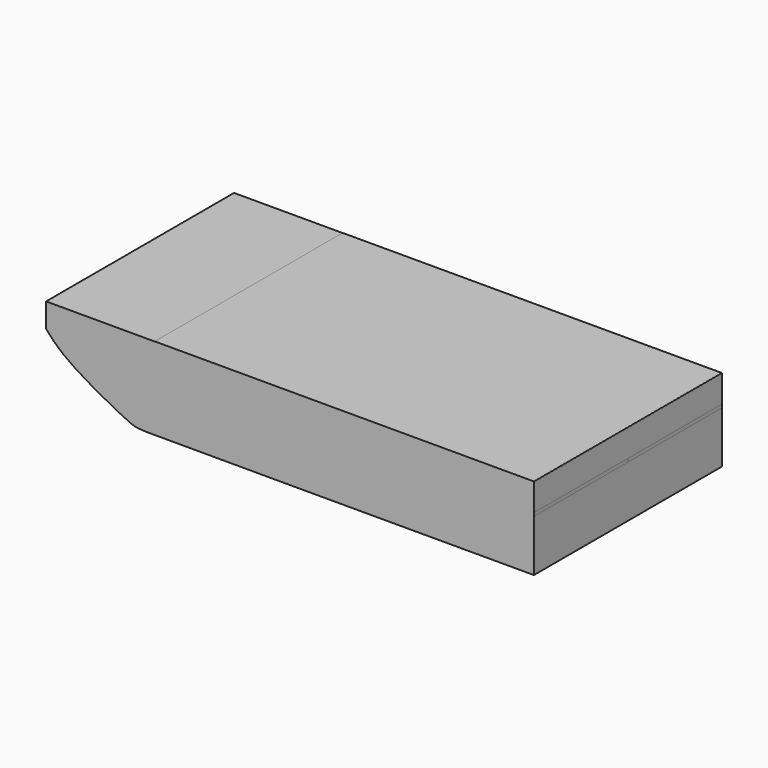
from build123d import *

# Parameters (mm, degrees)
F0_W     = 92
F0_H     = 57
F1_DEPTH = 20
F3_DEPTH = 28.5


with BuildPart() as f1:
    # F0 (on Top) → F1 (new body)
    with BuildSketch(Plane.XY):
        Rectangle(F0_W, F0_H)
    extrude(amount=F1_DEPTH)

    # F2 (on Front) → F3 (join, symmetric)
    with BuildSketch(Plane.XZ):
        with BuildLine():
            add(Edge.make_bspline(
                [(-72.352286854, 14.1225020504), (-70.7868680165, 12.1818560467), (-66.7235831643, 8.2633703724), (-51.3726170989, 0.0536119118), (-47.9178431553, -0.0501145074), (40.2776295905, -2.08522e-05), (46.0383226643, 0.002674896), (45.9645196982, 4.7811559883), (45.9713565107, 11.2640567196), (46.0139377281, 13.3675688924)],
                knots=[0, 0, 0, 0, 0.112628314, 0.2653870111, 0.3632089544, 0.7244735131, 0.8094160846, 0.8854591422, 1, 1, 1, 1], degree=3))
            Line((46.0139377281, 13.3675688924), (46.0139377281, 19.9693925679))
            Line((46.0139377281, 19.9693925679), (-72.352286854, 19.9693925679))
            Line((-72.352286854, 19.9693925679), (-72.352286854, 14.1225020504))
        make_face()
    extrude(amount=F3_DEPTH, both=True)


solid = f1.part
